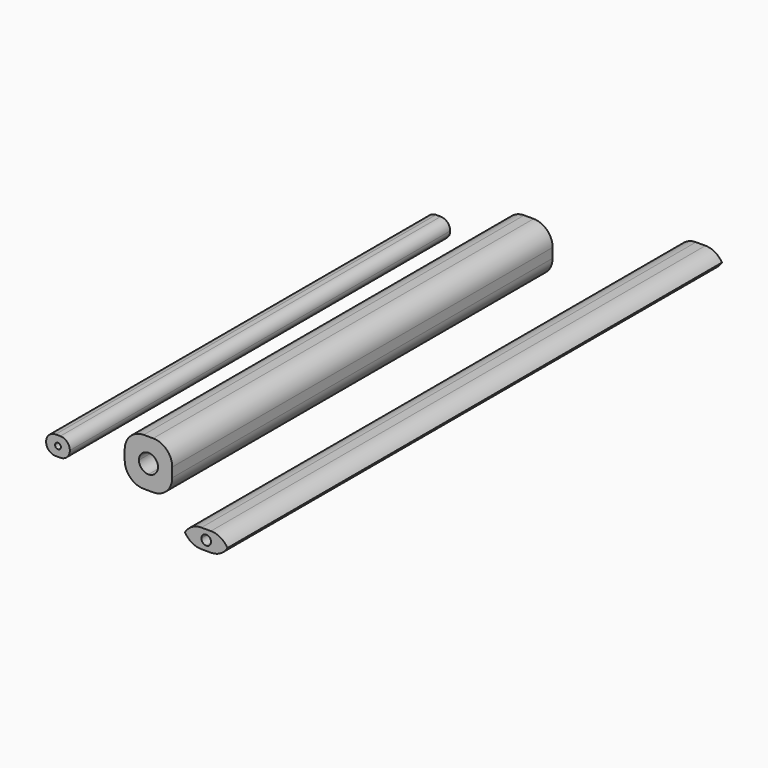
from build123d import *

# Parameters (mm, degrees)
F0_W         = 6.35
F0_H         = 127
F1_DEPTH     = 5.08
F2_R         = 2.53999
F4_DEPTH     = 12.7
F5_W         = 12.7
F5_H         = 127
F6_DEPTH     = 12.7
F7_R         = 5.08
F9_DEPTH     = 25.4
F10_W        = 12.7
F10_H        = 165.1
F11_DEPTH    = 5.08
F12_T1_DEPTH = 190.5
F14_DEPTH    = 25.4


# Not quite as in the source:
# - a fillet or chamfer that OpenCascade refuses, or shapes differently, is made with other operations: its cross-section is extruded or revolved along the edge and cut away or added
# - a fillet or chamfer is up to 0.001 mm smaller than in the source, because OpenCascade refuses the exact size


with BuildPart() as f1:
    # F0 (on Top) → F1 (new body)
    with BuildSketch(Plane.XY):
        with Locations((-44.3405173719, 7.7090010995)):
            Rectangle(F0_W, F0_H)
    extrude(amount=F1_DEPTH)

    # F2 (radius 2.54 in the source; OpenCascade refuses exactly that, so slightly less here)
    f2_edges = [f1.edges().sort_by_distance(p)[0] for p in [
        (-47.515517, 7.709001, 5.08),
        (-41.165517, 7.709001, 5.08),
        (-41.165517, 7.709001, 0),
        (-47.515517, 7.709001, 0),
    ]]
    fillet(f2_edges, radius=F2_R)

    # F3 (on face) → F4 (cut)
    with BuildSketch(Plane.XZ.offset(55.7909989005)):
        with BuildLine():
            Line((-45.1111345742, 2.54), (-44.3405173719, 2.54))
            Line((-44.3405173719, 2.54), (-44.3405173719, 3.3106172023))
            ThreePointArc((-44.3405173719, 3.3106172023), (-44.8854260214, 3.0849086495), (-45.1111345742, 2.54))
        make_face()
        with BuildLine():
            Line((-44.3405173719, 2.54), (-43.5699001695, 2.54))
            ThreePointArc((-43.5699001695, 2.54), (-43.7956087224, 3.0849086495), (-44.3405173719, 3.3106172023))
            Line((-44.3405173719, 3.3106172023), (-44.3405173719, 2.54))
        make_face()
        with BuildLine():
            ThreePointArc((-44.3405173719, 1.7693827977), (-43.7956087224, 1.9950913505), (-43.5699001695, 2.54))
            Line((-43.5699001695, 2.54), (-44.3405173719, 2.54))
            Line((-44.3405173719, 2.54), (-44.3405173719, 1.7693827977))
        make_face()
        with BuildLine():
            Line((-44.3405173719, 1.7693827977), (-44.3405173719, 2.54))
            Line((-44.3405173719, 2.54), (-45.1111345742, 2.54))
            ThreePointArc((-45.1111345742, 2.54), (-44.8854260214, 1.9950913505), (-44.3405173719, 1.7693827977))
        make_face()
    extrude(amount=-F4_DEPTH, mode=Mode.SUBTRACT)


with BuildPart() as f6:
    # F5 (on Top) → F6 (new body)
    with BuildSketch(Plane.XY):
        with Locations((-20.0740229338, 7.5928430158)):
            Rectangle(F5_W, F5_H)
    extrude(amount=F6_DEPTH)

    # F7
    f7_edges = [f6.edges().sort_by_distance(p)[0] for p in [
        (-26.424023, 7.592843, 12.7),
        (-13.724023, 7.592843, 12.7),
        (-13.724023, 7.592843, 0),
        (-26.424023, 7.592843, 0),
    ]]
    fillet(f7_edges, radius=F7_R)

    # F8 (on face) → F9 (cut)
    with BuildSketch(Plane.XZ.offset(55.9071569842)):
        with BuildLine():
            ThreePointArc((-17.5340229338, 6.35), (-18.2779717096, 8.1460512242), (-20.0740229338, 8.89))
            Line((-20.0740229338, 8.89), (-20.0740229338, 6.35))
            Line((-20.0740229338, 6.35), (-17.5340229338, 6.35))
        make_face()
        with BuildLine():
            Line((-20.0740229338, 6.35), (-20.0740229338, 8.89))
            ThreePointArc((-20.0740229338, 8.89), (-21.8700741581, 8.1460512242), (-22.6140229338, 6.35))
            Line((-22.6140229338, 6.35), (-20.0740229338, 6.35))
        make_face()
        with BuildLine():
            Line((-20.0740229338, 3.81), (-20.0740229338, 6.35))
            Line((-20.0740229338, 6.35), (-22.6140229338, 6.35))
            ThreePointArc((-22.6140229338, 6.35), (-21.8700741581, 4.5539487758), (-20.0740229338, 3.81))
        make_face()
        with BuildLine():
            Line((-17.5340229338, 6.35), (-20.0740229338, 6.35))
            Line((-20.0740229338, 6.35), (-20.0740229338, 3.81))
            ThreePointArc((-20.0740229338, 3.81), (-18.2779717096, 4.5539487758), (-17.5340229338, 6.35))
        make_face()
    extrude(amount=-F9_DEPTH, mode=Mode.SUBTRACT)


with BuildPart() as f11:
    # F10 (on Top) → F11 (new body)
    with BuildSketch(Plane.XY):
        with Locations((6.35, 12.8850169986)):
            Rectangle(F10_W, F10_H)
    extrude(amount=F11_DEPTH)

    # F12: fillet of radius 5.08 on 4 edges, made by hand

    # F12_s2 → F12_t1 (cut)
    with BuildSketch(Plane.XZ.offset(-108.1350169986)):
        with BuildLine():
            ThreePointArc((12.7, 0), (11.2121024484, 3.5921024484), (7.62, 5.08))
            Line((7.62, 5.08), (12.7, 5.08))
            Line((12.7, 5.08), (12.7, 0))
        make_face()
        with BuildLine():
            ThreePointArc((0, 0), (1.4878975516, 3.5921024484), (5.08, 5.08))
            Line((5.08, 5.08), (0, 5.08))
            Line((0, 5.08), (0, 0))
        make_face()
        with BuildLine():
            ThreePointArc((12.7, 5.08), (11.2121024484, 1.4878975516), (7.62, 0))
            Line((7.62, 0), (12.7, 0))
            Line((12.7, 0), (12.7, 5.08))
        make_face()
        with BuildLine():
            ThreePointArc((0, 5.08), (1.4878975516, 1.4878975516), (5.08, 0))
            Line((5.08, 0), (0, 0))
            Line((0, 0), (0, 5.08))
        make_face()
    extrude(amount=F12_T1_DEPTH, mode=Mode.SUBTRACT)

    # F13 (on face) → F14 (cut)
    with BuildSketch(Plane.XZ.offset(69.6649830014)):
        with BuildLine():
            ThreePointArc((7.6470044609, 2.54), (7.2671206496, 3.4571206496), (6.35, 3.8370044609))
            Line((6.35, 3.8370044609), (6.35, 2.54))
            Line((6.35, 2.54), (7.6470044609, 2.54))
        make_face()
        with BuildLine():
            Line((6.35, 2.54), (6.35, 3.8370044609))
            ThreePointArc((6.35, 3.8370044609), (5.4328793504, 3.4571206496), (5.0529955391, 2.54))
            Line((5.0529955391, 2.54), (6.35, 2.54))
        make_face()
        with BuildLine():
            Line((6.35, 1.2429955391), (6.35, 2.54))
            Line((6.35, 2.54), (5.0529955391, 2.54))
            ThreePointArc((5.0529955391, 2.54), (5.4328793504, 1.6228793504), (6.35, 1.2429955391))
        make_face()
        with BuildLine():
            Line((7.6470044609, 2.54), (6.35, 2.54))
            Line((6.35, 2.54), (6.35, 1.2429955391))
            ThreePointArc((6.35, 1.2429955391), (7.2671206496, 1.6228793504), (7.6470044609, 2.54))
        make_face()
    extrude(amount=-F14_DEPTH, mode=Mode.SUBTRACT)


solid = Compound([f1.part, f6.part, f11.part])
